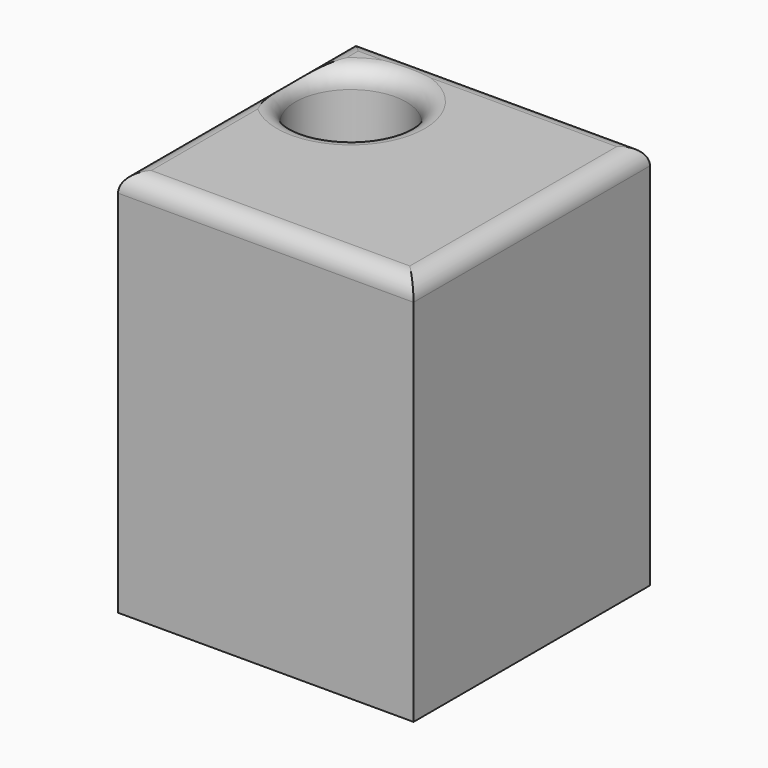
from build123d import *

# Parameters (mm, degrees)
F0_W        = 80
F0_H        = 80
F1_DEPTH    = 80
F2_DEPTH    = 25
F3_R        = 15
F4_DEPTH    = 105.001
F5_T1_DEPTH = 105
F5_T3_DEPTH = 105


# Not quite as in the source:
# - a fillet or chamfer that OpenCascade refuses, or shapes differently, is made with other operations: its cross-section is extruded or revolved along the edge and cut away or added


with BuildPart() as f1:
    # F0 (on Top) → F1 (new body)
    with BuildSketch(Plane.XY):
        with Locations((-101.8917422961, 32.1563994512)):
            Rectangle(F0_W, F0_H)
    extrude(amount=F1_DEPTH)

    # F2 (add): a face of the model
    f2_faces = [f1.faces().sort_by_distance(p)[0] for p in [
        (-101.8917422961, 32.1563994512, 80),
    ]]
    extrude(f2_faces, amount=F2_DEPTH)

    # F3 (on face) → F4 (cut, through all)
    with BuildSketch(Plane.XY.offset(105)):
        with Locations((-123.7266734242, 48.2279583812)):
            Circle(F3_R)
    extrude(amount=-F4_DEPTH, mode=Mode.SUBTRACT)

    # F5: fillet of radius 5 on 5 edges, made by hand

    # F5_s2 → F5_t1 (cut)
    with BuildSketch(Plane.YZ.offset(-154.3917422961)):
        with BuildLine():
            ThreePointArc((72.1563994512, 100), (70.6919333571, 103.5355339059), (67.1563994512, 105))
            Line((67.1563994512, 105), (72.1563994512, 105))
            Line((72.1563994512, 105), (72.1563994512, 100))
        make_face()
        with BuildLine():
            ThreePointArc((-2.8436005488, 105), (-6.3791344547, 103.5355339059), (-7.8436005488, 100))
            Line((-7.8436005488, 100), (-7.8436005488, 105))
            Line((-7.8436005488, 105), (-2.8436005488, 105))
        make_face()
    extrude(amount=F5_T1_DEPTH, mode=Mode.SUBTRACT)

    # F5_s4 → F5_t3 (cut)
    with BuildSketch(Plane.XZ.offset(-84.6563994512)):
        with BuildLine():
            ThreePointArc((-61.8917422961, 100), (-63.3562083901, 103.5355339059), (-66.8917422961, 105))
            Line((-66.8917422961, 105), (-61.8917422961, 105))
            Line((-61.8917422961, 105), (-61.8917422961, 100))
        make_face()
        with BuildLine():
            ThreePointArc((-136.8917422961, 105), (-140.427276202, 103.5355339059), (-141.8917422961, 100))
            Line((-141.8917422961, 100), (-141.8917422961, 105))
            Line((-141.8917422961, 105), (-136.8917422961, 105))
        make_face()
    extrude(amount=F5_T3_DEPTH, mode=Mode.SUBTRACT)

    # F5_s5 → F5_t6 (revolve, cut)
    with BuildSketch(Plane.XZ.offset(-48.2279583812)):
        with BuildLine():
            ThreePointArc((-103.7266734242, 105), (-107.2622073302, 103.5355339059), (-108.7266734242, 100))
            Line((-108.7266734242, 100), (-108.7266734242, 105))
            Line((-108.7266734242, 105), (-103.7266734242, 105))
        make_face()
    revolve(axis=Axis((-123.7266734242, 48.2279583812, 105), (0, 0, 1)), mode=Mode.SUBTRACT)


solid = f1.part
